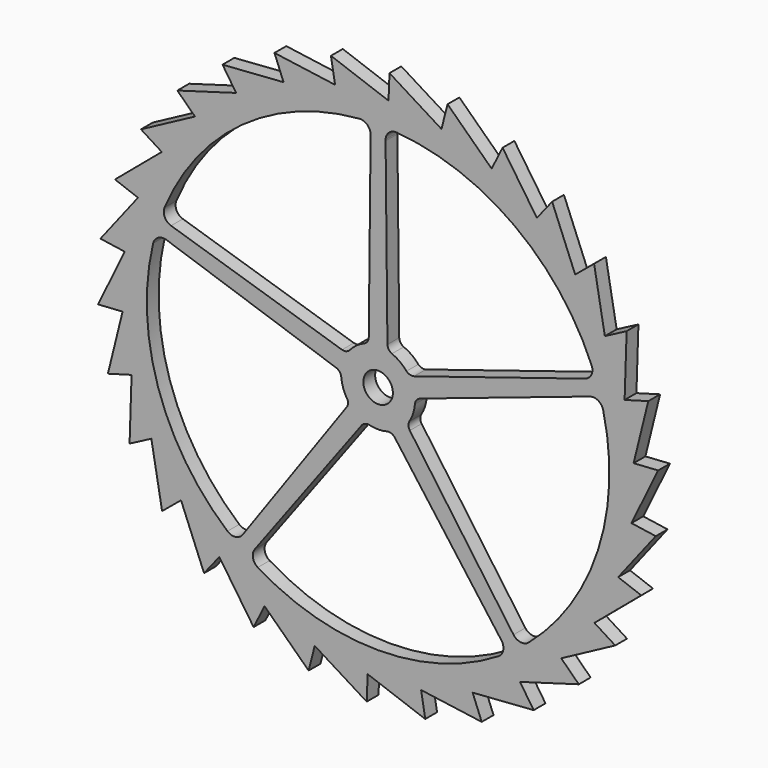
from build123d import *

# Parameters (mm, degrees)
F0_R     = 3
F1_DEPTH = 3


# Not quite as in the source:
# - ends of sketch curves that miss each other by under 0.0002 mm in the source are joined


with BuildPart() as f1:
    # F0 (on Front) → F1 (new body)
    with BuildSketch(Plane.XZ):
        with BuildLine():
            Line((-54.9035550344, -15.4022894368), (-50.0970420264, -14.0523310253))
            ThreePointArc((-50.0970420264, -14.0523310253), (-51.2908672182, -8.7471555647), (-51.9241410289, -3.346315858))
            Line((-51.9241410289, -3.346315858), (-54.9035550344, -15.4022894368))
        make_face()
        with BuildLine():
            Line((-50.5014645894, -26.4808034175), (-46.078343983, -24.1598005565))
            ThreePointArc((-46.078343983, -24.1598005565), (-48.3503436649, -19.2173511497), (-50.0935968915, -14.0645987898))
            Line((-50.0935968915, -14.0645987898), (-50.5014645894, -26.4808034175))
        make_face()
        with BuildLine():
            Line((-40.0472224692, -33.2111693559), (-40.0453648746, -33.2096278115))
            ThreePointArc((-40.0453648746, -33.2096278115), (-43.2978694534, -28.8447489774), (-46.0762579844, -24.1637757408))
            Line((-46.0762579844, -24.1637757408), (-43.8922178089, -36.4019792199))
            Line((-43.8922178089, -36.4019792199), (-40.0472224692, -33.2111693559))
        make_face()
        with BuildLine():
            ThreePointArc((-37.213042666, 36.354113843), (19.5968885399, 48.1537005723), (51.9680282572, 0.0007375898))
            ThreePointArc((51.9680282572, 0.0007375898), (17.6216901599, -48.9108992815), (-40.0453648746, -33.2096278115))
            Line((-40.0453648746, -33.2096278115), (-40.0472224692, -33.2111693559))
            Line((-40.0472224692, -33.2111693559), (-35.3646704919, -44.7322138543))
            Line((-35.3646704919, -44.7322138543), (-32.2671041994, -40.8117113592))
            Line((-32.2671041994, -40.8117113592), (-25.291517376, -51.1074360943))
            Line((-25.291517376, -51.1074360943), (-23.0767586415, -46.6285857397))
            Line((-23.0767586415, -46.6285857397), (-14.1130035885, -55.2490181363))
            Line((-14.1130035885, -55.2490181363), (-12.8778479963, -50.4075671746))
            Line((-12.8778479963, -50.4075671746), (-2.3176838225, -56.9759529715))
            Line((-2.3176838225, -56.9759529715), (-2.1161135989, -51.9834960417))
            Line((-2.1161135989, -51.9834960417), (9.578929848, -56.2127652609))
            Line((9.578929848, -56.2127652609), (8.738105117, -51.2874966872))
            Line((8.738105117, -51.2874966872), (21.0568983194, -52.9928099697))
            Line((21.0568983194, -52.9928099697), (19.2104267092, -48.3499876228))
            Line((19.2104267092, -48.3499876228), (31.614579292, -47.456814595))
            Line((31.614579292, -47.456814595), (28.8431604724, -43.2993520904))
            Line((28.8431604724, -43.2993520904), (40.7905514459, -39.8467286995))
            Line((40.7905514459, -39.8467286995), (37.2153097181, -36.3563270982))
            Line((37.2153097181, -36.3563270982), (48.1837807669, -30.495149554))
            Line((48.1837807669, -30.495149554), (43.9609713502, -27.8243561548))
            Line((43.9609713502, -27.8243561548), (53.4711476569, -19.810786041))
            Line((53.4711476569, -19.810786041), (48.7853275862, -18.0763273313))
            Line((48.7853275862, -18.0763273313), (56.4215688113, -8.2605961153))
            Line((56.4215688113, -8.2605961153), (51.4775309087, -7.5382762637))
            Line((51.4775309087, -7.5382762637), (56.9060966679, 3.6506214993))
            Line((56.9060966679, 3.6506214993), (51.9199191138, 3.3292336493))
            Line((51.9199191138, 3.3292336493), (54.9035550344, 15.4022894368))
            Line((54.9035550344, 15.4022894368), (50.0931577143, 14.0512400765))
            Line((50.0931577143, 14.0512400765), (50.5014645894, 26.4808034175))
            Line((50.5014645894, 26.4808034175), (46.0770849491, 24.1591398869))
            Line((46.0770849491, 24.1591398869), (43.8922178089, 36.4019792199))
            Line((43.8922178089, 36.4019792199), (40.0472224692, 33.2111693559))
            Line((40.0472224692, 33.2111693559), (35.3646704919, 44.7322138543))
            Line((35.3646704919, 44.7322138543), (32.2671041994, 40.8117113592))
            Line((32.2671041994, 40.8117113592), (25.291517376, 51.1074360943))
            Line((25.291517376, 51.1074360943), (23.0767586415, 46.6285857397))
            Line((23.0767586415, 46.6285857397), (14.1130035885, 55.2490181363))
            Line((14.1130035885, 55.2490181363), (12.8778479963, 50.4075671746))
            Line((12.8778479963, 50.4075671746), (2.3176838225, 56.9759529715))
            Line((2.3176838225, 56.9759529715), (2.1161135989, 51.9834960417))
            Line((2.1161135989, 51.9834960417), (-9.578929848, 56.2127652609))
            Line((-9.578929848, 56.2127652609), (-8.738105117, 51.2874966872))
            Line((-8.738105117, 51.2874966872), (-21.0568983194, 52.9928099697))
            Line((-21.0568983194, 52.9928099697), (-19.2104267092, 48.3499876228))
            Line((-19.2104267092, 48.3499876228), (-31.614579292, 47.456814595))
            Line((-31.614579292, 47.456814595), (-28.8431604724, 43.2993520904))
            Line((-28.8431604724, 43.2993520904), (-40.7905514459, 39.8467286995))
            Line((-40.7905514459, 39.8467286995), (-37.2153097181, 36.3563270982))
            Line((-37.2153097181, 36.3563270982), (-37.213042666, 36.354113843))
        make_face()
        with BuildLine():
            ThreePointArc((-51.9252180927, -3.329575199), (-51.9892512273, 2.1081313753), (-51.4850447931, 7.5227900813))
            Line((-51.4850447931, 7.5227900813), (-56.9060966679, -3.6506214993))
            Line((-56.9060966679, -3.6506214993), (-51.9252180927, -3.329575199))
        make_face()
        with BuildLine():
            ThreePointArc((-51.4826684815, 7.5390268588), (-50.4134868512, 12.8733028114), (-48.7928353928, 18.0666772584))
            Line((-48.7928353928, 18.0666772584), (-56.4215688113, 8.2605961153))
            Line((-56.4215688113, 8.2605961153), (-51.4826684815, 7.5390268588))
        make_face()
        with BuildLine():
            ThreePointArc((-48.7887845482, 18.0776069276), (-46.6313999834, 23.0765536675), (-43.9631489083, 27.8225217319))
            Line((-43.9631489083, 27.8225217319), (-53.4711476569, 19.810786041))
            Line((-53.4711476569, 19.810786041), (-48.7887845482, 18.0776069276))
        make_face()
        with BuildLine():
            ThreePointArc((-43.9616965875, 27.8248148444), (-40.810980226, 32.2663921953), (-37.213042666, 36.354113843))
            Line((-37.213042666, 36.354113843), (-37.2153097181, 36.3563270982))
            Line((-37.2153097181, 36.3563270982), (-48.1837807669, 30.495149554))
            Line((-48.1837807669, 30.495149554), (-43.9616965875, 27.8248148444))
        make_face()
        with BuildLine():
            ThreePointArc((-40.0453648746, -33.2096278115), (17.6216901599, -48.9108992815), (51.9680282572, 0.0007375898))
            ThreePointArc((51.9680282572, 0.0007375898), (19.5968885399, 48.1537005723), (-37.213042666, 36.354113843))
            ThreePointArc((-37.213042666, 36.354113843), (-40.810980226, 32.2663921953), (-43.9616965875, 27.8248148444))
            Line((-43.9616965875, 27.8248148444), (-43.9609713502, 27.8243561548))
            Line((-43.9609713502, 27.8243561548), (-43.9631489083, 27.8225217319))
            ThreePointArc((-43.9631489083, 27.8225217319), (-46.6313999834, 23.0765536675), (-48.7887845482, 18.0776069276))
            Line((-48.7887845482, 18.0776069276), (-48.7853275862, 18.0763273313))
            Line((-48.7853275862, 18.0763273313), (-48.7928353928, 18.0666772584))
            ThreePointArc((-48.7928353928, 18.0666772584), (-50.4134868512, 12.8733028114), (-51.4826684815, 7.5390268588))
            Line((-51.4826684815, 7.5390268588), (-51.4775309087, 7.5382762637))
            Line((-51.4775309087, 7.5382762637), (-51.4850447931, 7.5227900813))
            ThreePointArc((-51.4850447931, 7.5227900813), (-51.9892512273, 2.1081313753), (-51.9252180927, -3.329575199))
            Line((-51.9252180927, -3.329575199), (-51.9199191138, -3.3292336493))
            Line((-51.9199191138, -3.3292336493), (-51.9241410289, -3.346315858))
            ThreePointArc((-51.9241410289, -3.346315858), (-51.2908672182, -8.7471555647), (-50.0970420264, -14.0523310253))
            Line((-50.0970420264, -14.0523310253), (-50.0931577143, -14.0512400765))
            Line((-50.0931577143, -14.0512400765), (-50.0935968915, -14.0645987898))
            ThreePointArc((-50.0935968915, -14.0645987898), (-48.3503436649, -19.2173511497), (-46.078343983, -24.1598005565))
            Line((-46.078343983, -24.1598005565), (-46.0770849491, -24.1591398869))
            Line((-46.0770849491, -24.1591398869), (-46.0762579844, -24.1637757408))
            ThreePointArc((-46.0762579844, -24.1637757408), (-43.2978694534, -28.8447489774), (-40.0453648746, -33.2096278115))
        make_face()
        with BuildLine():
            ThreePointArc((-30.6087391151, -35.6778020758), (-44.7067731309, -14.5130968099), (-45.716604598, 10.8971285435))
            ThreePointArc((-45.716604598, 10.8971285435), (-44.6888266126, 12.2495178643), (-42.9970423633, 12.4016708018))
            Line((-42.9970423633, 12.4016708018), (-8.5374908198, 0.7549345664))
            ThreePointArc((-8.5374908198, 0.7549345664), (-7.802812606, 0.2334413444), (-7.4763562171, -0.606280922))
            ThreePointArc((-7.4763562171, -0.606280922), (-7.1023953356, -2.4207800492), (-6.295061591, -4.0882530021))
            ThreePointArc((-6.295061591, -4.0882530021), (-6.110368074, -4.8890528159), (-6.4203264896, -5.6501821199))
            Line((-6.4203264896, -5.6501821199), (-27.5220429881, -35.3008406001))
            ThreePointArc((-27.5220429881, -35.3008406001), (-28.982263813, -36.169997062), (-30.6087391151, -35.6778020758))
        make_face(mode=Mode.SUBTRACT)
        with BuildLine():
            ThreePointArc((-3.3140903569, -7.8390852899), (-2.605779553, -7.348009739), (-1.7449401376, -7.3054081862))
            ThreePointArc((-1.7449401376, -7.3054081862), (0.0953413286, -7.5106137979), (1.9298112192, -7.258690321))
            ThreePointArc((1.9298112192, -7.258690321), (2.7233576861, -7.359465878), (3.3639632378, -7.8385235312))
            Line((3.3639632378, -7.8385235312), (25.0458548563, -37.0762875112))
            ThreePointArc((25.0458548563, -37.0762875112), (25.4242166332, -38.7478039241), (24.4447545721, -40.15413917))
            ThreePointArc((24.4447545721, -40.15413917), (0, -47.0112198203), (-24.4447545721, -40.15413917))
            ThreePointArc((-24.4447545721, -40.15413917), (-25.4244419331, -38.7466486047), (-25.0444515303, -37.0743973345))
            Line((-25.0444515303, -37.0743973345), (-3.3140903569, -7.8390852899))
        make_face(mode=Mode.SUBTRACT)
        Circle(F0_R, mode=Mode.SUBTRACT)
        with BuildLine():
            ThreePointArc((6.4471741649, -5.6173093292), (6.1735472682, -4.8379856687), (6.3338513372, -4.0277266657))
            ThreePointArc((6.3338513372, -4.0277266657), (7.1180750013, -2.3740588492), (7.4784253342, -0.5796866358))
            ThreePointArc((7.4784253342, -0.5796866358), (7.7924795682, 0.2445578995), (8.501749914, 0.7689095872))
            Line((8.501749914, 0.7689095872), (43.0127487418, 12.3542340284))
            ThreePointArc((43.0127487418, 12.3542340284), (44.7033596143, 12.1990887403), (45.7287674683, 10.8460277972))
            ThreePointArc((45.7287674683, 10.8460277972), (44.6986623329, -14.5380772109), (30.6087391151, -35.6778020758))
            ThreePointArc((30.6087391151, -35.6778020758), (28.981088763, -36.1698532243), (27.5206712423, -35.2989108229))
            Line((27.5206712423, -35.2989108229), (6.4471741649, -5.6173093292))
        make_face(mode=Mode.SUBTRACT)
        with BuildLine():
            ThreePointArc((-3.8222602806, 46.8331002873), (-2.1987863566, 46.2693571068), (-1.5211456849, 44.6900290612))
            Line((-1.5211456849, 44.6900290612), (-1.8962351794, 8.3486142496))
            ThreePointArc((-1.8962351794, 8.3486142496), (-2.1672430487, 7.4877471123), (-2.8678543046, 6.9188170979))
            ThreePointArc((-2.8678543046, 6.9188170979), (-4.448699798, 6.0269148343), (-5.7689849741, 4.7813590646))
            ThreePointArc((-5.7689849741, 4.7813590646), (-6.4883786855, 4.349305408), (-7.327543237, 4.3500331389))
            Line((-7.327543237, 4.3500331389), (-42.0742299498, 15.2448326022))
            ThreePointArc((-42.0742299498, 15.2448326022), (-43.3514722345, 16.3633646212), (-43.3866659022, 18.060781228))
            ThreePointArc((-43.3866659022, 18.060781228), (-27.6429423876, 38.0001960459), (-3.8222602806, 46.8331002873))
        make_face(mode=Mode.SUBTRACT)
        with BuildLine():
            ThreePointArc((7.3223415791, 4.3754103913), (6.4925133297, 4.3634953347), (5.7728084591, 4.7767528711))
            ThreePointArc((5.7728084591, 4.7767528711), (4.4269848697, 6.0428535987), (2.8124529645, 6.9414852879))
            ThreePointArc((2.8124529645, 6.9414852879), (2.1677110719, 7.4862173416), (1.8968851416, 8.2856411552))
            Line((1.8968851416, 8.2856411552), (1.5221296421, 44.5946960866))
            ThreePointArc((1.5221296421, 44.5946960866), (1.51727433, 44.7174608453), (1.5195947017, 44.8402996661))
            ThreePointArc((1.5195947017, 44.8402996661), (2.223945132, 46.3120259473), (3.7686203119, 46.8374461259))
            ThreePointArc((3.7686203119, 46.8374461259), (3.7902743371, 46.8356991867), (3.8119275524, 46.8339422387))
            ThreePointArc((3.8119275524, 46.8339422387), (27.6368928258, 38.0045947169), (43.3848998793, 18.0650204541))
            ThreePointArc((43.3848998793, 18.0650204541), (43.3495674455, 16.3669469507), (42.0713630645, 15.2485125252))
            Line((42.0713630645, 15.2485125252), (7.3223415791, 4.3754103913))
        make_face(mode=Mode.SUBTRACT)
    extrude(amount=F1_DEPTH)


solid = f1.part
